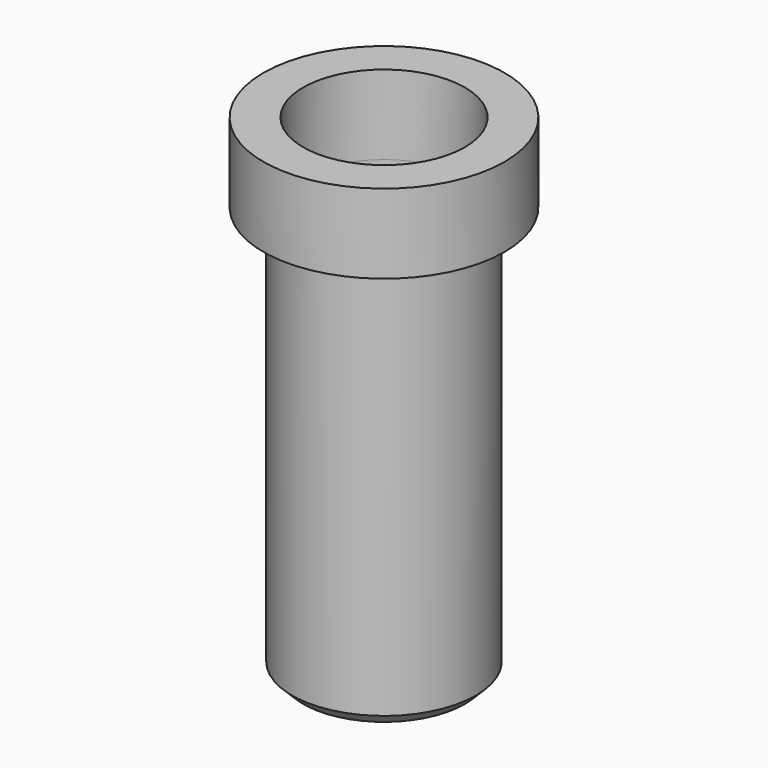
from build123d import *

# Parameters (mm, degrees)
F0_R     = 0.9652
F0_R_2   = 0.7366
F0_R_3   = 0.6477
F1_DEPTH = 0.635
F2_DEPTH = 3.3


# Not quite as in the source:
# - a fillet or chamfer that OpenCascade refuses, or shapes differently, is made with other operations: its cross-section is extruded or revolved along the edge and cut away or added


with BuildPart() as f1:
    # F0 (on Top) → F1 (new body)
    with BuildSketch(Plane.XY):
        Circle(F0_R)
        Circle(F0_R_2, mode=Mode.SUBTRACT)
        Circle(F0_R_2)
        Circle(F0_R_3, mode=Mode.SUBTRACT)
    extrude(amount=F1_DEPTH)

    # F0 (on Top) → F2 (join)
    with BuildSketch(Plane.XY):
        Circle(F0_R_2)
        Circle(F0_R_3, mode=Mode.SUBTRACT)
    extrude(amount=-F2_DEPTH)

    # F3: chamfer of 0.1 on 1 edges, made by hand

    # F3_s1 → F3_t2 (revolve, cut)
    with BuildSketch(Plane.XZ):
        Polygon((0.6366, -3.3), (0.7366, -3.2), (0.7366, -3.3), align=None)
    revolve(axis=Axis((0, 0, -3.3), (0, 0, 1)), mode=Mode.SUBTRACT)


solid = f1.part
